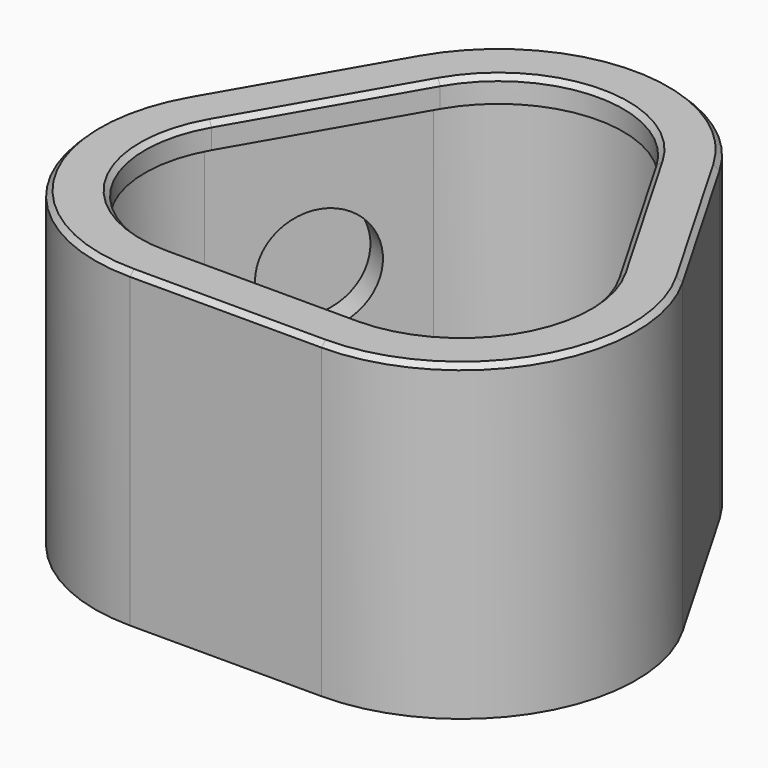
from build123d import *

# Parameters (mm, degrees)
F1_DEPTH        = 25
F3_START        = -0.65
F2_R            = 4.3
F3_DEPTH        = 2.15
F3_COPIES_COUNT = 3
F6_DEPTH        = 23
F8_DEPTH        = 2
F9_SIZE         = 0.6
F10_SIZE        = 0.4


# Not quite as in the source:
# - a pattern or mirror of a feature is missing from the dataset's text; its kind, count and spacing are read off the source's solid


with BuildPart() as f1:
    # F0 (on Top) → F1 (new body)
    with BuildSketch(Plane.XY):
        with BuildLine():
            ThreePointArc((7.6794919243, -4), (19.8038475773, 3), (19.8038475773, 17))
            Line((19.8038475773, 17), (12.124355653, 30.3012701892))
            ThreePointArc((12.124355653, 30.3012701892), (0, 37.3012701892), (-12.124355653, 30.3012701892))
            Line((-12.124355653, 30.3012701892), (-19.8038475773, 17))
            ThreePointArc((-19.8038475773, 17), (-19.8038475773, 3), (-7.6794919243, -4))
            Line((-7.6794919243, -4), (0, -4))
            Line((0, -4), (7.6794919243, -4))
        make_face()
        with BuildLine():
            Line((7.6794919243, 0), (0, 0))
            Line((0, 0), (-7.6794919243, 0))
            ThreePointArc((-7.6794919243, 0), (-16.3397459622, 5), (-16.3397459622, 15))
            Line((-16.3397459622, 15), (-8.6602540378, 28.3012701892))
            ThreePointArc((-8.6602540378, 28.3012701892), (0, 33.3012701892), (8.6602540378, 28.3012701892))
            Line((8.6602540378, 28.3012701892), (16.3397459622, 15))
            ThreePointArc((16.3397459622, 15), (16.3397459622, 5), (7.6794919243, 0))
        make_face(mode=Mode.SUBTRACT)
    extrude(amount=F1_DEPTH)

    # F2 (on face) → F3 (cut)
    with BuildSketch(Plane(origin=(-22.2141016151, 12.8253175473, 0), x_dir=(-0.5, -0.8660254038, 0), z_dir=(-0.8660254038, 0.5, 0)).offset(F3_START)):
        with Locations((-12.5, 12.5)):
            Circle(F2_R)
    f3 = extrude(amount=-F3_DEPTH, mode=Mode.SUBTRACT)

    # F3_copies: F3 ×3 about axis
    f3_copies_axis = Axis((0, 14.433757, 0), (0, 0, 1))
    for i in range(1, F3_COPIES_COUNT):
        add(f3.rotate(f3_copies_axis, i * 360 / F3_COPIES_COUNT), mode=Mode.SUBTRACT)

    # F5 (on face) → F6 (cut)
    with BuildSketch(Plane(origin=(0, 0, 0), x_dir=(1, 0, 0), z_dir=(0, 0, -1))):
        with BuildLine():
            Line((9.6994845224, -28.9012701892), (17.3789764467, -15.6))
            ThreePointArc((17.3789764467, -15.6), (17.3789764467, -4.4), (7.6794919243, 1.2))
            Line((7.6794919243, 1.2), (-7.6794919243, 1.2))
            ThreePointArc((-7.6794919243, 1.2), (-17.3789764467, -4.4), (-17.3789764467, -15.6))
            Line((-17.3789764467, -15.6), (-9.6994845224, -28.9012701892))
            ThreePointArc((-9.6994845224, -28.9012701892), (0, -34.5012701892), (9.6994845224, -28.9012701892))
        make_face()
    extrude(amount=-F6_DEPTH, mode=Mode.SUBTRACT)

    # F7 (on face) → F8 (cut)
    with BuildSketch(Plane(origin=(0, 0, 0), x_dir=(1, 0, 0), z_dir=(0, 0, -1))):
        with BuildLine():
            Line((11.0851251684, -29.7012701892), (18.7646170928, -16.4))
            ThreePointArc((18.7646170928, -16.4), (18.7646170928, -3.6), (7.6794919243, 2.8))
            Line((7.6794919243, 2.8), (-7.6794919243, 2.8))
            ThreePointArc((-7.6794919243, 2.8), (-18.7646170928, -3.6), (-18.7646170928, -16.4))
            Line((-18.7646170928, -16.4), (-11.0851251684, -29.7012701892))
            ThreePointArc((-11.0851251684, -29.7012701892), (0, -36.1012701892), (11.0851251684, -29.7012701892))
        make_face()
    extrude(amount=-F8_DEPTH, mode=Mode.SUBTRACT)

    # F9
    f9_edges = [f1.edges().sort_by_distance(p)[0] for p in [
        (0, 34.50127, 2),
        (13.53923, 22.250635, 2),
        (17.378976, 4.4, 2),
        (0, -1.2, 2),
        (-17.378976, 4.4, 2),
        (-13.53923, 22.250635, 2),
    ]]
    chamfer(f9_edges, length=F9_SIZE)

    # F10
    f10_edges = [f1.edges().sort_by_distance(p)[0] for p in [
        (19.803848, 3, 25),
        (12.5, 21.650635, 25),
        (0, -4, 25),
        (-19.803848, 3, 25),
        (-15.964102, 23.650635, 25),
        (15.964102, 23.650635, 25),
        (0, 37.30127, 25),
        (16.339746, 5, 25),
        (0, 0, 25),
        (-16.339746, 5, 25),
        (-12.5, 21.650635, 25),
        (0, 33.30127, 25),
    ]]
    chamfer(f10_edges, length=F10_SIZE)


solid = f1.part
